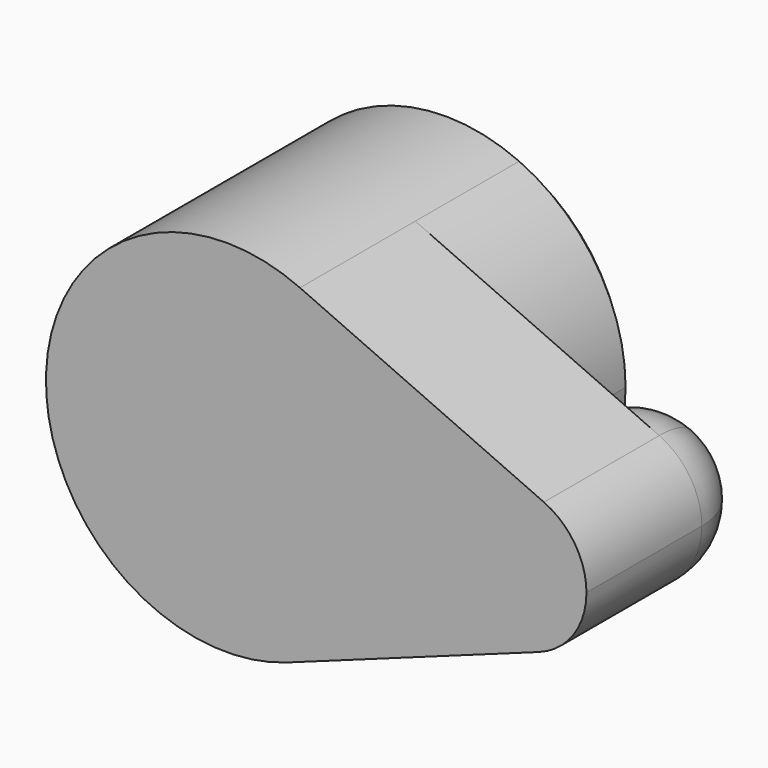
from build123d import *
from build123d import SkipClean  # not in build123d's __all__

# Parameters (mm, degrees)
F1_DEPTH = 25.4
F2_DEPTH = 25.4
F3_DEPTH = 12.7
F4_R     = 12.69999
F5_SIZE  = 2.54


# Not quite as in the source:
# - a fillet or chamfer is up to 0.001 mm smaller than in the source, because OpenCascade refuses the exact size
# - after a boolean that leaves OpenCascade's solid faulty, fix() repairs it


with BuildPart() as f1:
    # F0 (on Front) → F1 (new body)
    with BuildSketch(Plane.XZ):
        with BuildLine():
            ThreePointArc((-51.8046888554, -8.5958305632), (-36.6155359926, 3.0241505339), (-30.8559403173, 21.2604161342))
            ThreePointArc((-30.8559403173, 21.2604161342), (-35.9540680262, 38.515566188), (-49.6112287191, 50.2293645183))
            ThreePointArc((-49.6112287191, 50.2293645183), (-94.3338910639, 22.443480552), (-51.8046888554, -8.5958305632))
        make_face()
        with BuildLine():
            ThreePointArc((-49.6112287191, 50.2293645183), (-35.9540680262, 38.515566188), (-30.8559403173, 21.2604161342))
            ThreePointArc((-30.8559403173, 21.2604161342), (-36.6155359926, 3.0241505339), (-51.8046888554, -8.5958305632))
            Line((-51.8046888554, -8.5958305632), (-7.5207185378, 7.4250143868))
            ThreePointArc((-7.5207185378, 7.4250143868), (-24.5323994212, 19.8407388329), (-6.6433344833, 30.9550924194))
            Line((-6.6433344833, 30.9550924194), (-49.6112287191, 50.2293645183))
        make_face()
        with BuildLine():
            ThreePointArc((0.8587808774, 19.3675130658), (-1.1804702061, 26.2695730873), (-6.6433344833, 30.9550924194))
            ThreePointArc((-6.6433344833, 30.9550924194), (-24.5323994212, 19.8407388329), (-7.5207185378, 7.4250143868))
            ThreePointArc((-7.5207185378, 7.4250143868), (-1.4450573927, 12.0730068257), (0.8587808774, 19.3675130658))
        make_face()
    extrude(amount=F1_DEPTH)

    # F0 (on Front) → F2 (join)
    with BuildSketch(Plane.XZ):
        with BuildLine():
            ThreePointArc((-51.8046888554, -8.5958305632), (-36.6155359926, 3.0241505339), (-30.8559403173, 21.2604161342))
            ThreePointArc((-30.8559403173, 21.2604161342), (-35.9540680262, 38.515566188), (-49.6112287191, 50.2293645183))
            ThreePointArc((-49.6112287191, 50.2293645183), (-94.3338910639, 22.443480552), (-51.8046888554, -8.5958305632))
        make_face()
    with SkipClean():  # cleaning this boolean's faces spoils the solid; the shape is the same uncleaned
        extrude(amount=-F2_DEPTH)

    # F0 (on Front) → F3 (join)
    with BuildSketch(Plane.XZ):
        with BuildLine():
            ThreePointArc((0.8587808774, 19.3675130658), (-1.1804702061, 26.2695730873), (-6.6433344833, 30.9550924194))
            ThreePointArc((-6.6433344833, 30.9550924194), (-24.5323994212, 19.8407388329), (-7.5207185378, 7.4250143868))
            ThreePointArc((-7.5207185378, 7.4250143868), (-1.4450573927, 12.0730068257), (0.8587808774, 19.3675130658))
        make_face()
    extrude(amount=-F3_DEPTH)

    add(f1.part.fix(), mode=Mode.REPLACE)

    # F4 (radius 12.7 in the source; OpenCascade refuses exactly that, so slightly less here)
    f4_edges = [f1.edges().sort_by_distance(p)[0] for p in [
        (-16.16172, 12.7, 31.310012),
    ]]
    fillet(f4_edges, radius=F4_R)

    # F5
    f5_edges = [f1.edges().sort_by_distance(p)[0] for p in [
        (-73.407192, 25.4, 51.116663),
    ]]
    chamfer(f5_edges, length=F5_SIZE)


solid = f1.part
